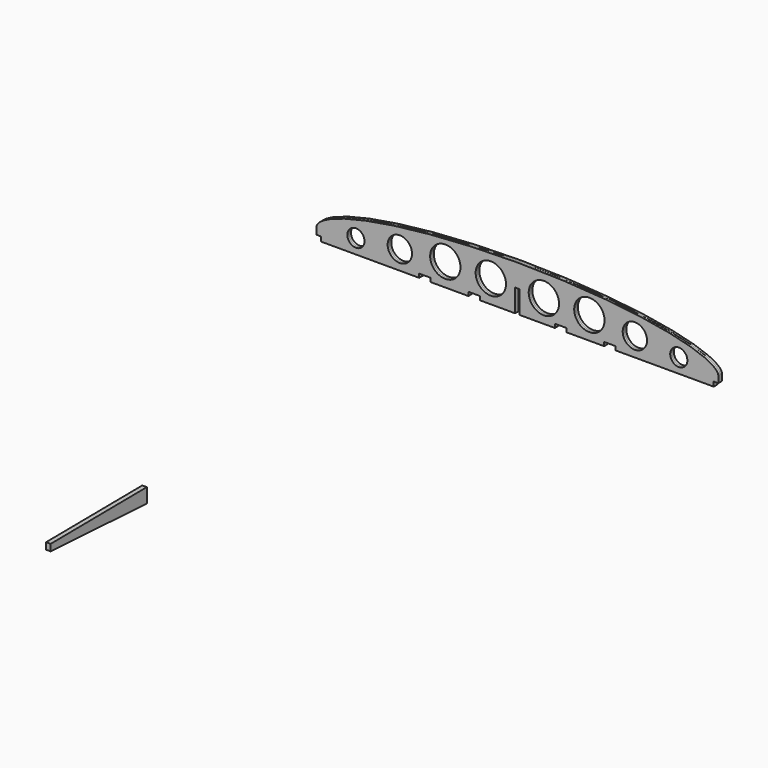
from build123d import *

# Parameters (mm, degrees)
F13_R     = 11.3226827756
F13_R_2   = 16.0602215827
F13_R_3   = 20
F14_DEPTH = 3
F16_DEPTH = 3


# Not quite as in the source:
# - ends of sketch curves that miss each other by under 0.0002 mm in the source are joined
# - the dataset's text gives a spline's control points without its knots; the knots are read off the source's solid


with BuildPart() as f14:
    # F13 (on plane+point) → F14 (new body, symmetric)
    with BuildSketch(Plane.XZ.offset(-900)):
        with BuildLine():
            add(Edge.make_bspline(
                [(0, 65.0000017214), (-16.8132716262, 65.0000017214), (-50.4436594842, 64.3772177187), (-99.3025047051, 61.6918414949), (-137.3620190284, 58.0943852226), (-165.4098100123, 54.4631954875), (-185.0417959114, 51.3800009944), (-203.0635795445, 47.9551169207), (-219.2641655203, 44.2095883028), (-233.4245941815, 40.1700613915), (-245.3115843014, 35.8773618028), (-253.1066747999, 32.1477127494), (-257.9267935516, 29.159352958), (-260.7953195745, 26.9605190172), (-262.8893252044, 24.8705031892), (-264.217468598, 22.9832715337), (-264.8761935592, 21.3845998162), (-265.0000017214, 20.4687501614), (-265.0000017214, 20)],
                knots=[0, 0, 0, 0, 0.125, 0.25, 0.375, 0.4375, 0.5, 0.5625, 0.625, 0.6875, 0.75, 0.8125, 0.84375, 0.875, 0.90625, 0.9375, 0.96875, 1, 1, 1, 1], degree=3))
            Line((-265.0000017214, 20), (-265.0000017214, 14))
            Line((-265.0000017214, 14), (-265.0000017214, 11))
            Line((-265.0000017214, 11), (-259.0000017214, 11))
            Line((-259.0000017214, 11), (-259.0000017214, 5))
            Line((-259.0000017214, 5), (-129.5000008607, 5))
            Line((-129.5000008607, 5), (-129.5000008607, 10))
            Line((-129.5000008607, 10), (-114.5000008607, 10))
            Line((-114.5000008607, 10), (-114.5000008607, 5))
            Line((-114.5000008607, 5), (-64.5000008607, 5))
            Line((-64.5000008607, 5), (-64.5000008607, 10))
            Line((-64.5000008607, 10), (-49.5000008607, 10))
            Line((-49.5000008607, 10), (-49.5000008607, 5))
            Line((-49.5000008607, 5), (-3, 5))
            Line((-3, 5), (-3, 35))
            Line((-3, 35), (0, 35))
            Line((0, 35), (3, 35))
            Line((3, 35), (3, 5))
            Line((3, 5), (49.5000008607, 5))
            Line((49.5000008607, 5), (49.5000008607, 10))
            Line((49.5000008607, 10), (64.5000008607, 10))
            Line((64.5000008607, 10), (64.5000008607, 5))
            Line((64.5000008607, 5), (114.5000008607, 5))
            Line((114.5000008607, 5), (114.5000008607, 10))
            Line((114.5000008607, 10), (129.5000008607, 10))
            Line((129.5000008607, 10), (129.5000008607, 5))
            Line((129.5000008607, 5), (259.0000017214, 5))
            Line((259.0000017214, 5), (259.0000017214, 11))
            Line((259.0000017214, 11), (265.0000017214, 11))
            Line((265.0000017214, 11), (265.0000017214, 14))
            Line((265.0000017214, 14), (265.0000017214, 20))
            add(Edge.make_bspline(
                [(0, 65.0000017214), (16.8132716049, 65), (50.4436594217, 64.377215998), (99.3025045792, 61.6918397777), (137.3620188431, 58.0943835108), (165.4098097701, 54.4631937831), (185.0417956199, 51.3799992976), (203.0635791939, 47.9551152349), (219.2641650964, 44.2095866337), (233.4245936626, 40.1700597488), (245.3115836539, 35.8773602052), (253.1066739993, 32.1477112211), (257.9267925836, 29.1593515313), (260.7953184537, 26.9605177048), (262.8893239024, 24.8705020511), (264.217467098, 22.9832706618), (264.876191886, 21.3845993314), (265, 20.46875), (265.0000017214, 20)],
                knots=[0, 0, 0, 0, 0.125, 0.25, 0.375, 0.4375, 0.5, 0.5625, 0.625, 0.6875, 0.75, 0.8125, 0.84375, 0.875, 0.90625, 0.9375, 0.96875, 1, 1, 1, 1], degree=3))
        make_face()
        with Locations((-212.9026800394, 24.1589043289)):
            Circle(F13_R, mode=Mode.SUBTRACT)
        with Locations((-154.9880802631, 30.0264377147)):
            Circle(F13_R_2, mode=Mode.SUBTRACT)
        with Locations((-95, 35)):
            Circle(F13_R_3, mode=Mode.SUBTRACT)
        with Locations((-35, 35)):
            Circle(F13_R_3, mode=Mode.SUBTRACT)
        with Locations((35, 35)):
            Circle(F13_R_3, mode=Mode.SUBTRACT)
        with Locations((95, 35)):
            Circle(F13_R_3, mode=Mode.SUBTRACT)
        with Locations((212.9026800394, 24.1589043289)):
            Circle(F13_R, mode=Mode.SUBTRACT)
        with Locations((154.9880802631, 30.0264377147)):
            Circle(F13_R_2, mode=Mode.SUBTRACT)
    extrude(amount=F14_DEPTH, both=True)


with BuildPart() as f16:
    # F15 (on Right) → F16 (new body, symmetric)
    with BuildSketch(Plane.YZ):
        Polygon((123.8436113754, 53.5422320686), (123.8436113754, 44.7781579091), (282.4514806271, 35.8825288713), (282.4514806271, 55.0000010676), align=None)
    extrude(amount=F16_DEPTH, both=True)


solid = Compound([f14.part, f16.part])
